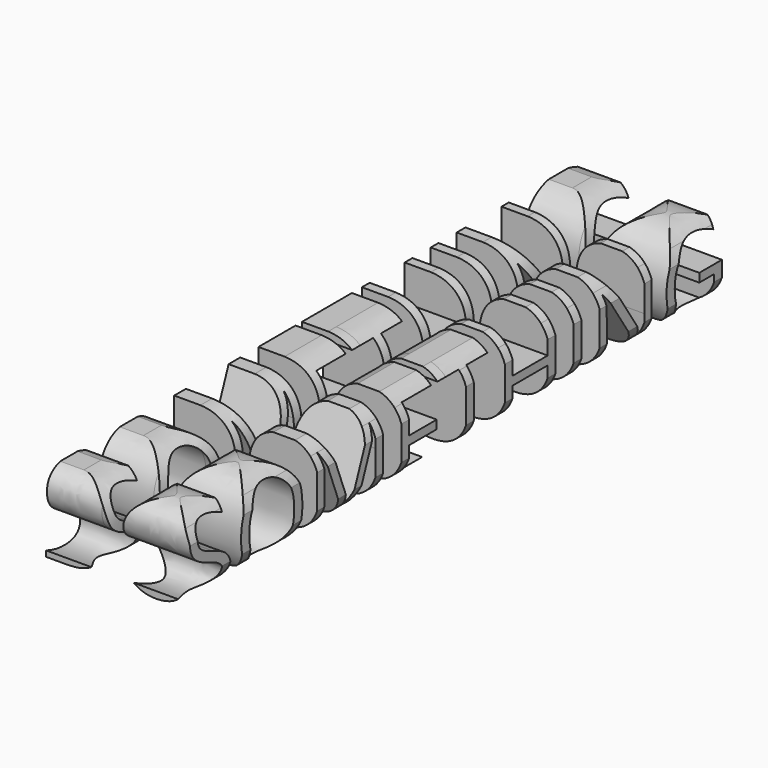
from build123d import *

# Parameters (mm, degrees)
F1_TEXT_SIZE  = 74.0833360598
F2_DEPTH      = 35.56
F2_DEPTH_BACK = 55.88
F0_W          = 111.4380322397
F0_H          = 65.8611282706
F3_DEPTH      = 254
F3_DEPTH_BACK = 254


# Not quite as in the source:
# - Text() gives the source's letters only with a copy of the font that has no kerning and outlines rounded to 1/6400 em; it was checked with that copy


with BuildPart() as f2:
    # F1 (on Right) → F2 (new body, two sides)
    with BuildSketch(Plane.YZ) as f2_sk:
        with Locations((-213.5510039531, -32.9305650666)):
            Text('SOMETHING', F1_TEXT_SIZE, font='Open Sans', text_align=(TextAlign.LEFT, TextAlign.BOTTOM))
    extrude(amount=-F2_DEPTH)
    extrude(f2_sk.sketch, amount=F2_DEPTH_BACK)

    # F0 (on Front) → F3 (cut, two sides)
    with BuildSketch(Plane.XZ) as f3_sk:
        with Locations((15.5261997133, -4.5076049864)):
            Rectangle(F0_W, F0_H)
        with BuildLine():
            add(Edge.make_bspline(
                [(-2.2491013713, 13.670010875), (4.0727907108, 7.3481187929), (4.0727907108, -4.0002395593)],
                knots=[0, 0, 0, 1, 1, 1], degree=2))
            add(Edge.make_bspline(
                [(4.0727907108, -4.0002395593), (4.0727907108, -16.1087238012), (-2.5006923348, -22.5162638708)],
                knots=[0, 0, 0, 1, 1, 1], degree=2))
            add(Edge.make_bspline(
                [(-2.5006923348, -22.5162638708), (-9.0741753803, -28.9238039404), (-21.418191588, -28.9238039404)],
                knots=[0, 0, 0, 1, 1, 1], degree=2))
            Line((-21.418191588, -28.9238039404), (-34.97198562, -28.9238039404))
            Line((-34.97198562, -28.9238039404), (-34.97198562, 19.9919029571))
            Line((-34.97198562, 19.9919029571), (-19.9835877963, 19.9919029571))
            add(Edge.make_bspline(
                [(-19.9835877963, 19.9919029571), (-8.5709934534, 19.9919029571), (-2.2491013713, 13.670010875)],
                knots=[0, 0, 0, 1, 1, 1], degree=2))
        make_face(mode=Mode.SUBTRACT)
        with BuildLine():
            add(Edge.make_bspline(
                [(51.5217758212, 14.0714858167), (57.4421929616, 7.3802367883), (57.4421929616, -4.3963615018)],
                knots=[0, 0, 0, 1, 1, 1], degree=2))
            add(Edge.make_bspline(
                [(57.4421929616, -4.3963615018), (57.4421929616, -16.1408417965), (51.5003638243, -22.8695618195)],
                knots=[0, 0, 0, 1, 1, 1], degree=2))
            add(Edge.make_bspline(
                [(51.5003638243, -22.8695618195), (45.5585346871, -29.5982818425), (34.9917142214, -29.5982818425)],
                knots=[0, 0, 0, 1, 1, 1], degree=2))
            add(Edge.make_bspline(
                [(34.9917142214, -29.5982818425), (24.1893617899, -29.5982818425), (18.3171216425, -22.9873278024)],
                knots=[0, 0, 0, 1, 1, 1], degree=2))
            add(Edge.make_bspline(
                [(18.3171216425, -22.9873278024), (12.4448814952, -16.3763737623), (12.4448814952, -4.3321255111)],
                knots=[0, 0, 0, 1, 1, 1], degree=2))
            add(Edge.make_bspline(
                [(12.4448814952, -4.3321255111), (12.4448814952, 7.6157687541), (18.3331806402, 14.1892517996)],
                knots=[0, 0, 0, 1, 1, 1], degree=2))
            add(Edge.make_bspline(
                [(18.3331806402, 14.1892517996), (24.2214797852, 20.7627348451), (35.0559502121, 20.7627348451)],
                knots=[0, 0, 0, 1, 1, 1], degree=2))
            add(Edge.make_bspline(
                [(35.0559502121, 20.7627348451), (45.6013586809, 20.7627348451), (51.5217758212, 14.0714858167)],
                knots=[0, 0, 0, 1, 1, 1], degree=2))
        make_face(mode=Mode.SUBTRACT)
    extrude(amount=-F3_DEPTH, mode=Mode.SUBTRACT)
    extrude(f3_sk.sketch, amount=F3_DEPTH_BACK, mode=Mode.SUBTRACT)


solid = f2.part
